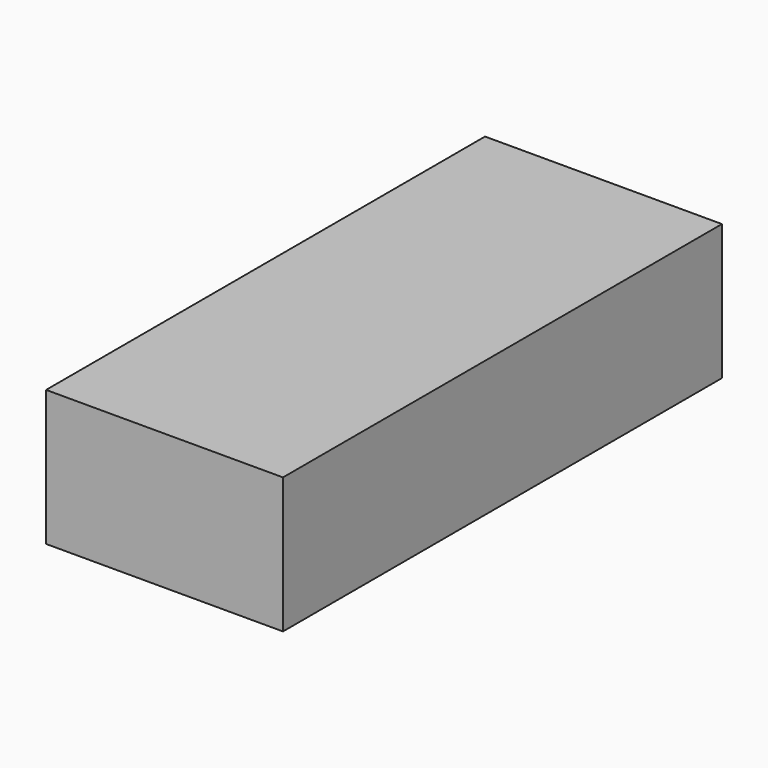
from build123d import *

# Parameters (mm, degrees)
F0_R     = 200
F1_DEPTH = 2200
F2_R     = 175
F3_DEPTH = 1050
F4_R     = 175
F5_DEPTH = 1050
F7_W     = 4317.6512718201
F7_H     = 2472.1434116364
F8_DEPTH = 10000


with BuildPart() as f1:
    # F0 (on Front) → F1 (new body)
    with BuildSketch(Plane.XZ):
        Circle(F0_R)
    extrude(amount=F1_DEPTH)

    # F2 (on Front) → F3 (cut)
    with BuildSketch(Plane.XZ):
        Circle(F2_R)
    extrude(amount=F3_DEPTH, mode=Mode.SUBTRACT)

    # F4 (on face) → F5 (cut)
    with BuildSketch(Plane.XZ.offset(2200)):
        Circle(F4_R)
    extrude(amount=-F5_DEPTH, mode=Mode.SUBTRACT)


with BuildPart() as f8:
    # F7 (on offset) → F8 (new body)
    with BuildSketch(Plane.XZ.offset(-2000)):
        Rectangle(F7_W, F7_H)
    extrude(amount=F8_DEPTH)


solid = Compound([f1.part, f8.part])
